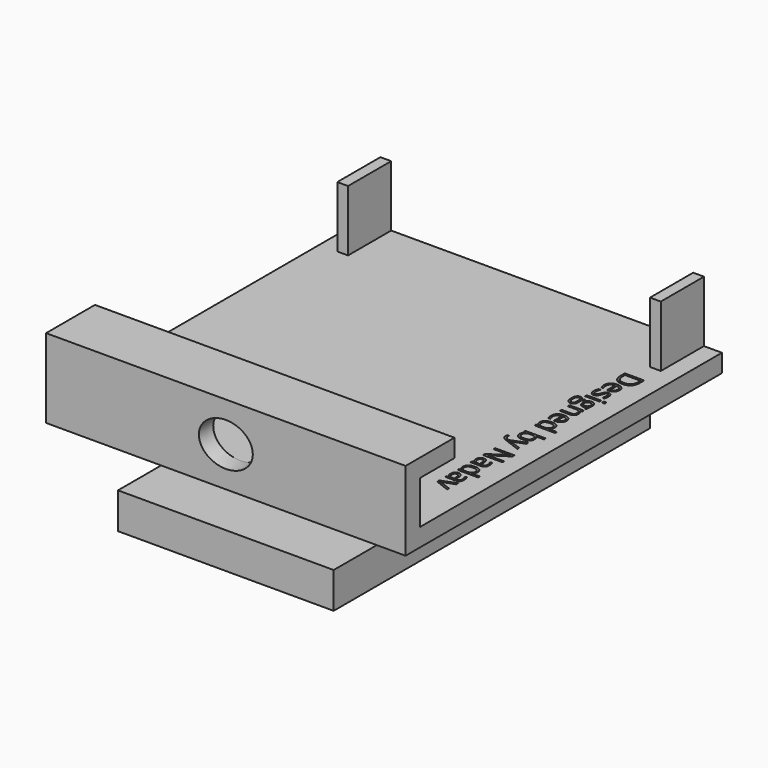
from build123d import *

# Parameters (mm, degrees)
F0_W          = 60
F0_H          = 110
F1_DEPTH      = 10
F2_W          = 40
F2_H          = 40
F3_DEPTH      = 10
F4_W          = 100
F4_H          = 110
F4_W_2        = 40
F4_H_2        = 40
F5_DEPTH      = 5
F6_W          = 3
F6_H          = 15
F6_W_2        = 100
F6_H_2        = 5
F7_DEPTH      = 17
F9_DEPTH      = 12
F10_DEPTH     = 25
F11_TEXT_SIZE = 7.5248551915
F12_DEPTH     = 1


# Not quite as in the source:
# - Text() gives the source's letters only with a copy of the font that has no kerning and outlines rounded to 1/6400 em; it was checked with that copy


with BuildPart() as f1:
    # F0 (on Top) → F1 (new body)
    with BuildSketch(Plane.XY):
        Rectangle(F0_W, F0_H)
    extrude(amount=F1_DEPTH)

    # F2 (on face) → F3 (join)
    with BuildSketch(Plane.XY.offset(10)):
        Rectangle(F2_W, F2_H)
    extrude(amount=F3_DEPTH)

    # F4 (on face) → F5 (join)
    with BuildSketch(Plane.XY.offset(20)):
        Rectangle(F4_W, F4_H)
        Rectangle(F4_W_2, F4_H_2, mode=Mode.SUBTRACT)
        Rectangle(F4_W_2, F4_H_2)
    extrude(amount=F5_DEPTH)

    # F6 (on face) → F7 (join)
    with BuildSketch(Plane.XY.offset(25)):
        with Locations((-43.5, 47.5)):
            Rectangle(F6_W, F6_H)
        with Locations((43.5, 47.5)):
            Rectangle(F6_W, F6_H)
        with Locations((0, -52.5)):
            Rectangle(F6_W_2, F6_H_2)
    extrude(amount=F7_DEPTH)

    # F8 (on face) → F9 (join)
    with BuildSketch(Plane(origin=(0, -50, 0), x_dir=(-1, 0, 0), z_dir=(0, 1, 0))):
        Polygon((-2.19e-08, 37), (50, 37), (50, 42), (-50, 42), (-50, 37), align=None)
    extrude(amount=F9_DEPTH)

    # F8 (on face) → F10 (cut)
    with BuildSketch(Plane(origin=(0, -50, 0), x_dir=(-1, 0, 0), z_dir=(0, 1, 0))):
        with BuildLine():
            add(Edge.make_bspline(
                [(-3.19e-08, 25), (7.499999995, 24.9999999744), (7.5, 30.999999996), (7.500000005, 37.0000000175), (-2.19e-08, 37)],
                knots=[1.5707963225, 1.5707963225, 1.5707963225, 3.1415926529, 3.1415926529, 4.7123889833, 4.7123889833, 4.7123889833], degree=2, weights=[1, 0.7071067799, 1, 0.7071067799, 1]))
            add(Edge.make_bspline(
                [(-2.19e-08, 37), (-7.5, 36.9999999825), (-7.5, 31)],
                knots=[4.7123889833, 4.7123889833, 4.7123889833, 6.2831853072, 6.2831853072, 6.2831853072], degree=2, weights=[1, 0.7071067822, 1]))
            add(Edge.make_bspline(
                [(-7.5, 31), (-7.5, 25.0000000256), (-3.19e-08, 25)],
                knots=[0, 0, 0, 1.5707963225, 1.5707963225, 1.5707963225], degree=2, weights=[1, 0.7071067827, 1]))
        make_face()
    extrude(amount=-F10_DEPTH, mode=Mode.SUBTRACT)

    # F11 (on face) → F12 (cut)
    with BuildSketch(Plane.XY.offset(25)):
        with Locations(Location((39.5821042621, 35), (0, 0, -90))):
            Text('Designed by Nadav', F11_TEXT_SIZE, font='Open Sans', text_align=(TextAlign.LEFT, TextAlign.BOTTOM))
    extrude(amount=-F12_DEPTH, mode=Mode.SUBTRACT)


solid = f1.part
